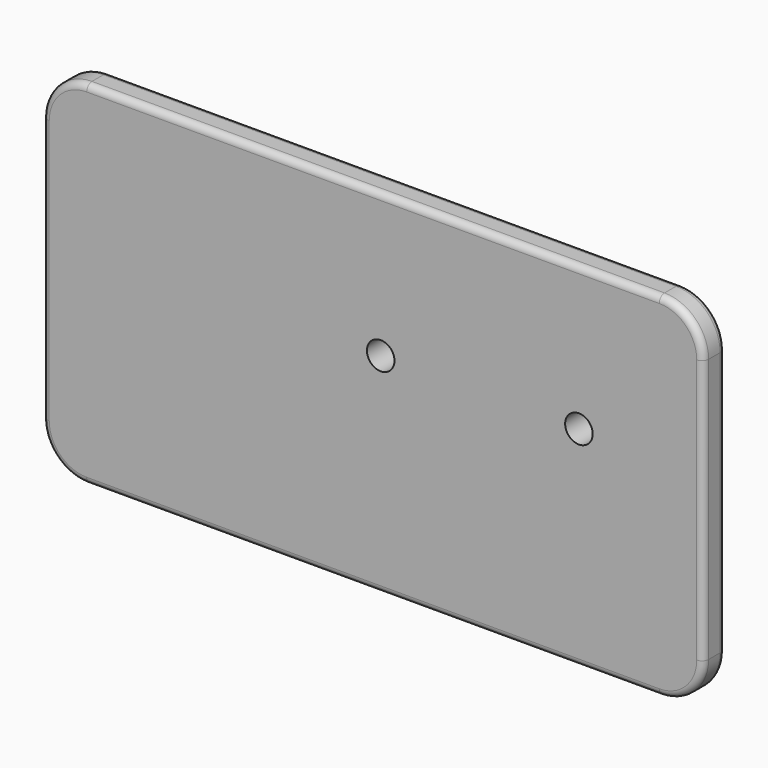
from build123d import *

# Parameters (mm, degrees)
F0_W     = 76.2
F0_H     = 40.64
F0_R     = 1.5875
F1_DEPTH = 3.175
F2_R     = 5.08
F3_R     = 0.762


# Not quite as in the source:
# - a feature names something its author has since deleted; it is built from what else it names


with BuildPart() as f1:
    # F0 (on Front) → F1 (new body)
    with BuildSketch(Plane.XZ):
        with Locations((-5.08, -3.81)):
            Rectangle(F0_W, F0_H)
        with Locations((-4.191, 0)):
            Circle(F0_R, mode=Mode.SUBTRACT)
        with Locations((18.669, 0)):
            Circle(F0_R, mode=Mode.SUBTRACT)
    extrude(amount=F1_DEPTH)

    # F2
    f2_edges = [f1.edges().sort_by_distance(p)[0] for p in [
        (-43.18, -1.5875, -24.13),
        (33.02, -1.5875, 16.51),
        (33.02, -1.5875, -24.13),
        (-43.18, -1.5875, 16.51),
    ]]
    fillet(f2_edges, radius=F2_R)

    # F3
    f3_edges = [f1.edges().sort_by_distance(p)[0] for p in [
        (-5.08, 0, -24.13),
        (-5.08, -3.175, -24.13),
        (-43.18, -3.175, -3.81),
        (-43.18, 0, -3.81),
        (-41.692102, 0, -22.642102),
        (31.532102, 0, -22.642102),
        (33.02, 0, -3.81),
        (-41.692102, 0, 15.022102),
        (31.532102, 0, 15.022102),
        (-5.08, 0, 16.51),
        (-41.692102, -3.175, -22.642102),
        (31.532102, -3.175, -22.642102),
        (33.02, -3.175, -3.81),
        (-41.692102, -3.175, 15.022102),
        (31.532102, -3.175, 15.022102),
        (-5.08, -3.175, 16.51),
    ]]
    fillet(f3_edges, radius=F3_R)


solid = f1.part
